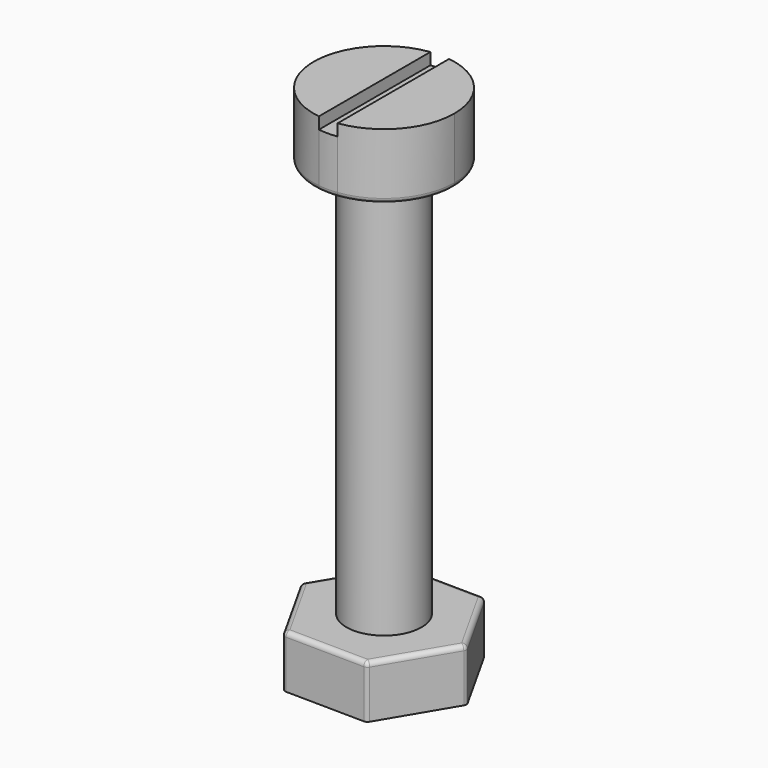
from build123d import *

# Parameters (mm, degrees)
F1_DEPTH      = 2.25
F2_R          = 1.6
F3_DEPTH      = 22
F3_DEPTH_BACK = 0.5
F5_DEPTH      = 2.8
F6_R          = 0.2
F6_2_R        = 0.2
F7_DEPTH      = 0.5


# Not quite as in the source:
# - a feature names something its author has since deleted; it is built from what else it names


with BuildPart() as f1:
    # F0 (on Top) → F1 (new body)
    with BuildSketch(Plane.XY):
        Polygon((3.5792652324, -0.0468372692), (1.8301948812, 3.0763159835), (-1.7490703512, 3.1231532527), (-3.5792652324, 0.0468372692), (-1.8301948812, -3.0763159835), (1.7490703512, -3.1231532527), align=None)
    extrude(amount=F1_DEPTH)

    # F6#2
    f6_2_edges = [f1.edges().sort_by_distance(p)[0] for p in [
        (2.664168, -1.584995, 2.25),
        (2.70473, 1.514739, 2.25),
        (-0.040562, -3.099735, 2.25),
        (-2.70473, -1.514739, 2.25),
        (0.040562, 3.099735, 2.25),
        (-2.664168, 1.584995, 2.25),
        (-1.830195, -3.076316, 1.125),
        (1.74907, -3.123153, 1.125),
        (3.579265, -0.046837, 1.125),
        (-3.579265, 0.046837, 1.125),
        (1.830195, 3.076316, 1.125),
        (-1.74907, 3.123153, 1.125),
    ]]
    fillet(f6_2_edges, radius=F6_2_R)


with BuildPart() as f3:
    # F2 (on Top) → F3 (new body, two sides)
    with BuildSketch(Plane.XY) as f3_sk:
        Circle(F2_R)
    extrude(amount=F3_DEPTH)
    extrude(f3_sk.sketch, amount=-F3_DEPTH_BACK)

    # F4 (on face) → F5 (join)
    with BuildSketch(Plane.XY.offset(22)):
        with BuildLine():
            ThreePointArc((0.4, -2.9732137495), (2.2583179581, -1.9748417658), (3, 0))
            ThreePointArc((3, 0), (2.2583179581, 1.9748417658), (0.4, 2.9732137495))
            Line((0.4, 2.9732137495), (0.4, -2.9732137495))
        make_face()
        with BuildLine():
            Line((0.4, -2.9732137495), (0.4, 2.9732137495))
            ThreePointArc((0.4, 2.9732137495), (0, 3), (-0.4, 2.9732137495))
            Line((-0.4, 2.9732137495), (-0.4, -2.9732137495))
            ThreePointArc((-0.4, -2.9732137495), (0, -3), (0.4, -2.9732137495))
        make_face()
        with BuildLine():
            Line((-0.4, -2.9732137495), (-0.4, 2.9732137495))
            ThreePointArc((-0.4, 2.9732137495), (-3, 0), (-0.4, -2.9732137495))
        make_face()
    extrude(amount=-F5_DEPTH)

    # F6
    f6_edges = [f3.edges().sort_by_distance(p)[0] for p in [
        (0.4, -2.973214, 19.2),
    ]]
    fillet(f6_edges, radius=F6_R)

    # F4 (on face) → F7 (cut)
    with BuildSketch(Plane.XY.offset(22)):
        with BuildLine():
            Line((0.4, 1.5491933385), (0.4, 2.9732137495))
            ThreePointArc((0.4, 2.9732137495), (0, 3), (-0.4, 2.9732137495))
            Line((-0.4, 2.9732137495), (-0.4, 1.5491933385))
            ThreePointArc((-0.4, 1.5491933385), (0, 1.6), (0.4, 1.5491933385))
        make_face()
        with BuildLine():
            Line((0.4, -1.5491933385), (0.4, 1.5491933385))
            ThreePointArc((0.4, 1.5491933385), (0, 1.6), (-0.4, 1.5491933385))
            Line((-0.4, 1.5491933385), (-0.4, -1.5491933385))
            ThreePointArc((-0.4, -1.5491933385), (0, -1.6), (0.4, -1.5491933385))
        make_face()
        with BuildLine():
            ThreePointArc((-0.4, -2.9732137495), (0, -3), (0.4, -2.9732137495))
            Line((0.4, -2.9732137495), (0.4, -1.5491933385))
            ThreePointArc((0.4, -1.5491933385), (0, -1.6), (-0.4, -1.5491933385))
            Line((-0.4, -1.5491933385), (-0.4, -2.9732137495))
        make_face()
    extrude(amount=-F7_DEPTH, mode=Mode.SUBTRACT)


solid = Compound([f1.part, f3.part])
